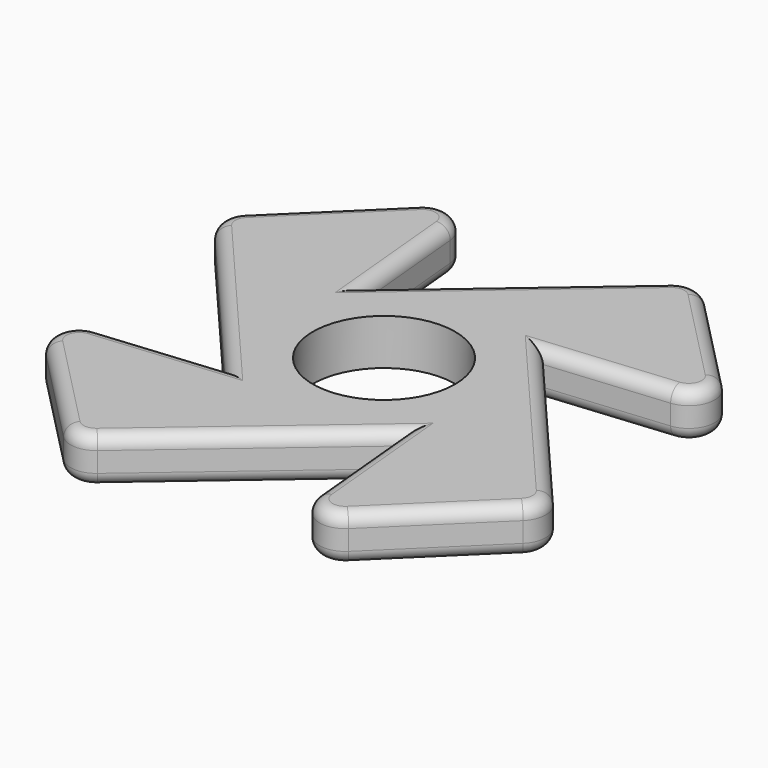
from build123d import *

# Parameters (mm, degrees)
F0_W         = 27.3088011891
F0_H         = 27.3088011891
F0_R         = 11
F1_DEPTH     = 7.1
F2_R         = 2
F3_T1_DEPTH  = 7.1
F3_T4_ANGLE  = 128.9490479257
F3_T6_ANGLE  = 128.9490479257
F3_T8_ANGLE  = 128.9490479257
F3_T10_ANGLE = 128.9490479257
F3_T12_ANGLE = 128.9490479257
F3_T14_ANGLE = 128.9490479257
F3_T16_ANGLE = 128.9490479257
F3_T18_ANGLE = 128.9490479257
F3_T20_ANGLE = 86.2266707628
F3_T22_ANGLE = 86.2266707628
F3_T24_ANGLE = 86.2266707628
F3_T26_ANGLE = 86.2266707628
F3_T28_ANGLE = 86.2266707628
F3_T30_ANGLE = 86.2266707628
F3_T32_ANGLE = 86.2266707628
F3_T34_ANGLE = 86.2266707628


# Not quite as in the source:
# - a fillet or chamfer that OpenCascade refuses, or shapes differently, is made with other operations: its cross-section is extruded or revolved along the edge and cut away or added


with BuildPart() as f1:
    # F0 (on Top) → F1 (new body)
    with BuildSketch(Plane.XY):
        Rectangle(F0_W, F0_H)
        Circle(F0_R, mode=Mode.SUBTRACT)
        Polygon((13.6544005945, 13.6544005945), (40.3753073238, 16.1683388102), (17.1169115879, 39.9823956144), (-13.6544005945, 13.6544005945), align=None)
        Polygon((16.1683388102, -40.3753073238), (39.9823956144, -17.1169115879), (13.6544005945, 13.6544005945), (13.6544005945, -13.6544005945), align=None)
        Polygon((-40.3753073238, -16.1683388102), (-17.1169115879, -39.9823956144), (13.6544005945, -13.6544005945), (-13.6544005945, -13.6544005945), align=None)
        Polygon((-13.6544005945, -13.6544005945), (-13.6544005945, 13.6544005945), (-16.1683388102, 40.3753073238), (-39.9823956144, 17.1169115879), align=None)
    extrude(amount=F1_DEPTH)

    # F2
    f2_edges = [f1.edges().sort_by_distance(p)[0] for p in [
        (-1.731255, -26.818398, 7.1),
        (14.91137, -27.014854, 7.1),
        (28.075367, -28.746109, 7.1),
        (26.818398, -1.731255, 7.1),
        (27.014854, 14.91137, 7.1),
        (28.746109, 28.075367, 7.1),
        (1.731255, 26.818398, 7.1),
        (-14.91137, 27.014854, 7.1),
        (-28.075367, 28.746109, 7.1),
        (-26.818398, 1.731255, 7.1),
        (-27.014854, -14.91137, 7.1),
        (-28.746109, -28.075367, 7.1),
        (-28.746109, -28.075367, 0),
        (-27.014854, -14.91137, 0),
        (-26.818398, 1.731255, 0),
        (-28.075367, 28.746109, 0),
        (-14.91137, 27.014854, 0),
        (1.731255, 26.818398, 0),
        (28.746109, 28.075367, 0),
        (27.014854, 14.91137, 0),
        (26.818398, -1.731255, 0),
        (28.075367, -28.746109, 0),
        (14.91137, -27.014854, 0),
        (-1.731255, -26.818398, 0),
    ]]
    fillet(f2_edges, radius=F2_R)

    # F3: fillet of radius 4 on 8 edges, made by hand

    # F3_s2 → F3_t1 (cut)
    with BuildSketch(Plane.XY):
        with BuildLine():
            ThreePointArc((37.3032935738, -19.7335012764), (38.5044476922, -17.050755387), (37.5477883044, -14.2714210172))
            Line((37.5477883044, -14.2714210172), (39.9823956144, -17.1169115879))
            Line((39.9823956144, -17.1169115879), (37.3032935738, -19.7335012764))
        make_face()
        with BuildLine():
            ThreePointArc((14.2714210172, 37.5477883044), (17.050755387, 38.5044476922), (19.7335012764, 37.3032935738))
            Line((19.7335012764, 37.3032935738), (17.1169115879, 39.9823956144))
            Line((17.1169115879, 39.9823956144), (14.2714210172, 37.5477883044))
        make_face()
        with BuildLine():
            ThreePointArc((-37.5477883044, 14.2714210172), (-38.5044476922, 17.050755387), (-37.3032935738, 19.7335012764))
            Line((-37.3032935738, 19.7335012764), (-39.9823956144, 17.1169115879))
            Line((-39.9823956144, 17.1169115879), (-37.5477883044, 14.2714210172))
        make_face()
        with BuildLine():
            ThreePointArc((-14.2714210172, -37.5477883044), (-17.050755387, -38.5044476922), (-19.7335012764, -37.3032935738))
            Line((-19.7335012764, -37.3032935738), (-17.1169115879, -39.9823956144))
            Line((-17.1169115879, -39.9823956144), (-14.2714210172, -37.5477883044))
        make_face()
        with BuildLine():
            ThreePointArc((15.383723208, -32.0355477412), (17.988166327, -35.4160328938), (22.1609818603, -34.5224925468))
            Line((22.1609818603, -34.5224925468), (16.1683388102, -40.3753073238))
            Line((16.1683388102, -40.3753073238), (15.383723208, -32.0355477412))
        make_face()
        with BuildLine():
            ThreePointArc((-34.5224925468, -22.1609818603), (-35.4160328938, -17.988166327), (-32.0355477412, -15.383723208))
            Line((-32.0355477412, -15.383723208), (-40.3753073238, -16.1683388102))
            Line((-40.3753073238, -16.1683388102), (-34.5224925468, -22.1609818603))
        make_face()
        with BuildLine():
            ThreePointArc((-22.1609818603, 34.5224925468), (-17.988166327, 35.4160328938), (-15.383723208, 32.0355477412))
            Line((-15.383723208, 32.0355477412), (-16.1683388102, 40.3753073238))
            Line((-16.1683388102, 40.3753073238), (-22.1609818603, 34.5224925468))
        make_face()
        with BuildLine():
            ThreePointArc((32.0355477412, 15.383723208), (35.4160328938, 17.988166327), (34.5224925468, 22.1609818603))
            Line((34.5224925468, 22.1609818603), (40.3753073238, 16.1683388102))
            Line((40.3753073238, 16.1683388102), (32.0355477412, 15.383723208))
        make_face()
    extrude(amount=F3_T1_DEPTH, mode=Mode.SUBTRACT)

    # F3_s3 → F3_t4 (revolve, cut)
    with BuildSketch(Plane(origin=(5.776383091, -5.914385352, 0), x_dir=(0, 0, 1), z_dir=(-0.6987111461, 0.7154038959, 0))):
        with BuildLine():
            ThreePointArc((0, 38.1816506997), (0.5857864376, 39.5958642621), (2, 40.1816506997))
            Line((2, 40.1816506997), (0, 40.1816506997))
            Line((0, 40.1816506997), (0, 38.1816506997))
        make_face()
    revolve(axis=Axis((31.6608769631, 19.3661372759, 0), (0, 0, -1)), revolution_arc=F3_T4_ANGLE, mode=Mode.SUBTRACT)

    # F3_s5 → F3_t6 (revolve, cut)
    with BuildSketch(Plane(origin=(33.1891022135, 3.1224745943, 0), x_dir=(0, 0, 1), z_dir=(-0.995603517, -0.0936676945, 0))):
        with BuildLine():
            ThreePointArc((7.1, 14.3153930302), (6.5142135624, 12.9011794678), (5.1, 12.3153930302))
            Line((5.1, 12.3153930302), (7.1, 12.3153930302))
            Line((7.1, 12.3153930302), (7.1, 14.3153930302))
        make_face()
    revolve(axis=Axis((31.6608769631, 19.3661372759, 7.1), (0, 0, 1)), revolution_arc=F3_T6_ANGLE, mode=Mode.SUBTRACT)

    # F3_s7 → F3_t8 (revolve, cut)
    with BuildSketch(Plane(origin=(5.914385352, 5.776383091, 0), x_dir=(0, 0, 1), z_dir=(-0.7154038959, -0.6987111461, 0))):
        with BuildLine():
            ThreePointArc((0, 38.1816506997), (0.5857864376, 39.5958642621), (2, 40.1816506997))
            Line((2, 40.1816506997), (0, 40.1816506997))
            Line((0, 40.1816506997), (0, 38.1816506997))
        make_face()
    revolve(axis=Axis((-19.3661372759, 31.6608769631, 0), (0, 0, -1)), revolution_arc=F3_T8_ANGLE, mode=Mode.SUBTRACT)

    # F3_s9 → F3_t10 (revolve, cut)
    with BuildSketch(Plane(origin=(-3.1224745943, 33.1891022135, 0), x_dir=(0, 0, 1), z_dir=(0.0936676945, -0.995603517, 0))):
        with BuildLine():
            ThreePointArc((7.1, 14.3153930302), (6.5142135624, 12.9011794678), (5.1, 12.3153930302))
            Line((5.1, 12.3153930302), (7.1, 12.3153930302))
            Line((7.1, 12.3153930302), (7.1, 14.3153930302))
        make_face()
    revolve(axis=Axis((-19.3661372759, 31.6608769631, 7.1), (0, 0, 1)), revolution_arc=F3_T10_ANGLE, mode=Mode.SUBTRACT)

    # F3_s11 → F3_t12 (revolve, cut)
    with BuildSketch(Plane(origin=(-5.776383091, 5.914385352, 0), x_dir=(0, 0, 1), z_dir=(0.6987111461, -0.7154038959, 0))):
        with BuildLine():
            ThreePointArc((0, 38.1816506997), (0.5857864376, 39.5958642621), (2, 40.1816506997))
            Line((2, 40.1816506997), (0, 40.1816506997))
            Line((0, 40.1816506997), (0, 38.1816506997))
        make_face()
    revolve(axis=Axis((-31.6608769631, -19.3661372759, 0), (0, 0, -1)), revolution_arc=F3_T12_ANGLE, mode=Mode.SUBTRACT)

    # F3_s13 → F3_t14 (revolve, cut)
    with BuildSketch(Plane(origin=(-33.1891022135, -3.1224745943, 0), x_dir=(0, 0, 1), z_dir=(0.995603517, 0.0936676945, 0))):
        with BuildLine():
            ThreePointArc((7.1, 14.3153930302), (6.5142135624, 12.9011794678), (5.1, 12.3153930302))
            Line((5.1, 12.3153930302), (7.1, 12.3153930302))
            Line((7.1, 12.3153930302), (7.1, 14.3153930302))
        make_face()
    revolve(axis=Axis((-31.6608769631, -19.3661372759, 7.1), (0, 0, 1)), revolution_arc=F3_T14_ANGLE, mode=Mode.SUBTRACT)

    # F3_s15 → F3_t16 (revolve, cut)
    with BuildSketch(Plane(origin=(-5.914385352, -5.776383091, 0), x_dir=(0, 0, 1), z_dir=(0.7154038959, 0.6987111461, 0))):
        with BuildLine():
            ThreePointArc((0, 38.1816506997), (0.5857864376, 39.5958642621), (2, 40.1816506997))
            Line((2, 40.1816506997), (0, 40.1816506997))
            Line((0, 40.1816506997), (0, 38.1816506997))
        make_face()
    revolve(axis=Axis((19.3661372759, -31.6608769631, 0), (0, 0, -1)), revolution_arc=F3_T16_ANGLE, mode=Mode.SUBTRACT)

    # F3_s17 → F3_t18 (revolve, cut)
    with BuildSketch(Plane(origin=(3.1224745943, -33.1891022135, 0), x_dir=(0, 0, 1), z_dir=(-0.0936676945, 0.995603517, 0))):
        with BuildLine():
            ThreePointArc((7.1, 14.3153930302), (6.5142135624, 12.9011794678), (5.1, 12.3153930302))
            Line((5.1, 12.3153930302), (7.1, 12.3153930302))
            Line((7.1, 12.3153930302), (7.1, 14.3153930302))
        make_face()
    revolve(axis=Axis((19.3661372759, -31.6608769631, 7.1), (0, 0, 1)), revolution_arc=F3_T18_ANGLE, mode=Mode.SUBTRACT)

    # F3_s19 → F3_t20 (revolve, cut)
    with BuildSketch(Plane(origin=(-26.7874807354, -22.9194210249, 0), x_dir=(0, 0, 1), z_dir=(0.7598348287, 0.6501161689, 0))):
        with BuildLine():
            ThreePointArc((0, 17.2520357401), (0.5857864376, 18.6662493025), (2, 19.2520357401))
            Line((2, 19.2520357401), (0, 19.2520357401))
            Line((0, 19.2520357401), (0, 17.2520357401))
        make_face()
    revolve(axis=Axis((-16.8718856926, -34.5084489895, 0), (0, 0, -1)), revolution_arc=F3_T20_ANGLE, mode=Mode.SUBTRACT)

    # F3_s21 → F3_t22 (revolve, cut)
    with BuildSketch(Plane(origin=(9.0126081794, -9.2279263615, 0), x_dir=(0, 0, 1), z_dir=(-0.6987111461, 0.7154038959, 0))):
        with BuildLine():
            ThreePointArc((7.1, -38.1816506997), (6.5142135624, -39.5958642621), (5.1, -40.1816506997))
            Line((5.1, -40.1816506997), (7.1, -40.1816506997))
            Line((7.1, -40.1816506997), (7.1, -38.1816506997))
        make_face()
    revolve(axis=Axis((-16.8718856926, -34.5084489895, 7.1), (0, 0, 1)), revolution_arc=F3_T22_ANGLE, mode=Mode.SUBTRACT)

    # F3_s23 → F3_t24 (revolve, cut)
    with BuildSketch(Plane(origin=(-22.9194210249, 26.7874807354, 0), x_dir=(0, 0, 1), z_dir=(0.6501161689, -0.7598348287, 0))):
        with BuildLine():
            ThreePointArc((0, 17.2520357401), (0.5857864376, 18.6662493025), (2, 19.2520357401))
            Line((2, 19.2520357401), (0, 19.2520357401))
            Line((0, 19.2520357401), (0, 17.2520357401))
        make_face()
    revolve(axis=Axis((-34.5084489895, 16.8718856926, 0), (0, 0, -1)), revolution_arc=F3_T24_ANGLE, mode=Mode.SUBTRACT)

    # F3_s25 → F3_t26 (revolve, cut)
    with BuildSketch(Plane(origin=(-9.2279263615, -9.0126081794, 0), x_dir=(0, 0, 1), z_dir=(0.7154038959, 0.6987111461, 0))):
        with BuildLine():
            ThreePointArc((7.1, -38.1816506997), (6.5142135624, -39.5958642621), (5.1, -40.1816506997))
            Line((5.1, -40.1816506997), (7.1, -40.1816506997))
            Line((7.1, -40.1816506997), (7.1, -38.1816506997))
        make_face()
    revolve(axis=Axis((-34.5084489895, 16.8718856926, 7.1), (0, 0, 1)), revolution_arc=F3_T26_ANGLE, mode=Mode.SUBTRACT)

    # F3_s27 → F3_t28 (revolve, cut)
    with BuildSketch(Plane(origin=(26.7874807354, 22.9194210249, 0), x_dir=(0, 0, 1), z_dir=(-0.7598348287, -0.6501161689, 0))):
        with BuildLine():
            ThreePointArc((0, 17.2520357401), (0.5857864376, 18.6662493025), (2, 19.2520357401))
            Line((2, 19.2520357401), (0, 19.2520357401))
            Line((0, 19.2520357401), (0, 17.2520357401))
        make_face()
    revolve(axis=Axis((16.8718856926, 34.5084489895, 0), (0, 0, -1)), revolution_arc=F3_T28_ANGLE, mode=Mode.SUBTRACT)

    # F3_s29 → F3_t30 (revolve, cut)
    with BuildSketch(Plane(origin=(-9.0126081794, 9.2279263615, 0), x_dir=(0, 0, 1), z_dir=(0.6987111461, -0.7154038959, 0))):
        with BuildLine():
            ThreePointArc((7.1, -38.1816506997), (6.5142135624, -39.5958642621), (5.1, -40.1816506997))
            Line((5.1, -40.1816506997), (7.1, -40.1816506997))
            Line((7.1, -40.1816506997), (7.1, -38.1816506997))
        make_face()
    revolve(axis=Axis((16.8718856926, 34.5084489895, 7.1), (0, 0, 1)), revolution_arc=F3_T30_ANGLE, mode=Mode.SUBTRACT)

    # F3_s31 → F3_t32 (revolve, cut)
    with BuildSketch(Plane(origin=(22.9194210249, -26.7874807354, 0), x_dir=(0, 0, 1), z_dir=(-0.6501161689, 0.7598348287, 0))):
        with BuildLine():
            ThreePointArc((0, 17.2520357401), (0.5857864376, 18.6662493025), (2, 19.2520357401))
            Line((2, 19.2520357401), (0, 19.2520357401))
            Line((0, 19.2520357401), (0, 17.2520357401))
        make_face()
    revolve(axis=Axis((34.5084489895, -16.8718856926, 0), (0, 0, -1)), revolution_arc=F3_T32_ANGLE, mode=Mode.SUBTRACT)

    # F3_s33 → F3_t34 (revolve, cut)
    with BuildSketch(Plane(origin=(9.2279263615, 9.0126081794, 0), x_dir=(0, 0, 1), z_dir=(-0.7154038959, -0.6987111461, 0))):
        with BuildLine():
            ThreePointArc((7.1, -38.1816506997), (6.5142135624, -39.5958642621), (5.1, -40.1816506997))
            Line((5.1, -40.1816506997), (7.1, -40.1816506997))
            Line((7.1, -40.1816506997), (7.1, -38.1816506997))
        make_face()
    revolve(axis=Axis((34.5084489895, -16.8718856926, 7.1), (0, 0, 1)), revolution_arc=F3_T34_ANGLE, mode=Mode.SUBTRACT)


solid = f1.part
